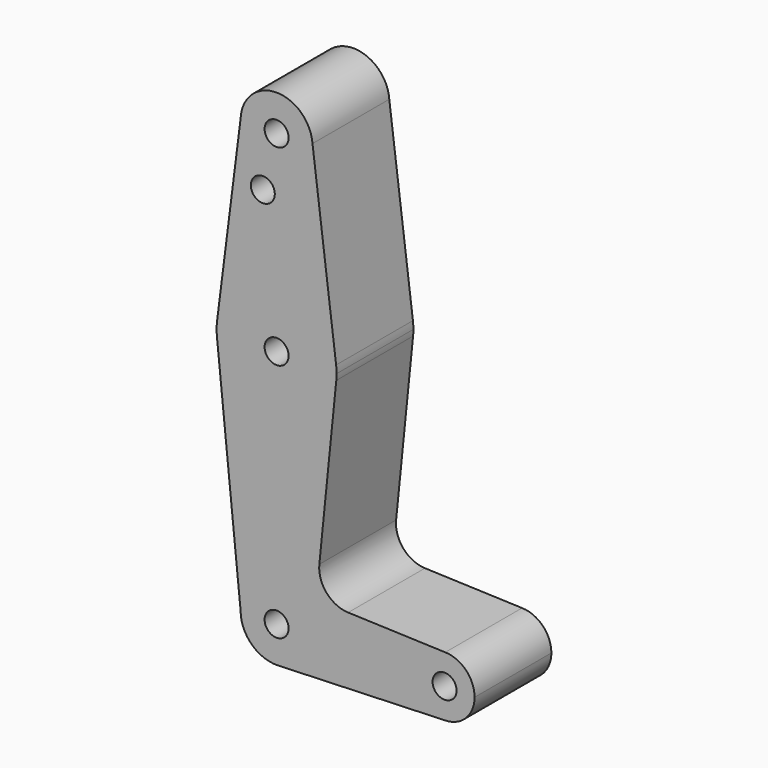
from build123d import *

# Parameters (mm, degrees)
F0_R     = 3.175
F1_DEPTH = 25.4


# Not quite as in the source:
# - a feature names something its author has since deleted; it is built from what else it names


with BuildPart() as f1:
    # F0 (on Front) → F1 (new body)
    with BuildSketch(Plane.XZ):
        with BuildLine():
            ThreePointArc((-9.5149138168, 114.7382237551), (-0.2191699059, 104.7775218797), (9.525, 114.3))
            ThreePointArc((9.525, 114.3), (9.5183168712, 114.6567477241), (9.4982768633, 115.0129948306))
            ThreePointArc((9.4982768633, 115.0129948306), (-0.1376371427, 123.8240055133), (-9.5149138168, 114.7382237551))
        make_face()
        with Locations((0, 114.3)):
            Circle(F0_R, mode=Mode.SUBTRACT)
        with BuildLine():
            ThreePointArc((9.4982768633, 115.0129948306), (9.5183168712, 114.6567477241), (9.525, 114.3))
            ThreePointArc((9.525, 114.3), (-0.2191699059, 104.7775218797), (-9.5149138168, 114.7382237551))
            Line((-9.5149138168, 114.7382237551), (-15.7492887561, 65.4938727833))
            ThreePointArc((-15.7492887561, 65.4938727833), (0.002863253, 79.3749997418), (15.7500069708, 65.4881914948))
            Line((15.7500069708, 65.4881914948), (9.4982768633, 115.0129948306))
        make_face()
        with Locations((-3.6479982082, 100.0252)):
            Circle(F0_R, mode=Mode.SUBTRACT)
        with BuildLine():
            ThreePointArc((15.875, 63.5), (15.8437209276, 64.4960583162), (15.7500069708, 65.4881914948))
            ThreePointArc((15.7500069708, 65.4881914948), (0.002863253, 79.3749997418), (-15.7492887561, 65.4938727833))
            ThreePointArc((-15.7492887561, 65.4938727833), (-15.8737601653, 63.698401651), (-15.7942028036, 61.9003804205))
            ThreePointArc((-15.7942028036, 61.9003804205), (0, 47.625), (15.7942028036, 61.9003804205))
            ThreePointArc((15.7942028036, 61.9003804205), (15.8547878338, 62.6991705884), (15.875, 63.5))
        make_face()
        with Locations((0, 63.5)):
            Circle(F0_R, mode=Mode.SUBTRACT)
        with BuildLine():
            ThreePointArc((15.7942028036, 61.9003804205), (0, 47.625), (-15.7942028036, 61.9003804205))
            Line((-15.7942028036, 61.9003804205), (-9.525, 0))
            ThreePointArc((-9.525, 0), (0, 9.525), (9.525, 0))
            ThreePointArc((9.525, 0), (6.854575784, -6.6136537422), (0.3406607199, -9.5189062016))
            Line((0.3406607199, -9.5189062016), (44.5449382907, -7.9369322141))
            ThreePointArc((44.5449382907, -7.9369322141), (36.5126173213, 0.0431562547), (44.6312377373, 7.9354306205))
            Line((44.6312377373, 7.9354306205), (18.9332319933, 8.8541850706))
            ThreePointArc((18.9332319933, 8.8541850706), (13.2249062601, 11.5746494613), (11.3075490968, 17.6003984343))
            Line((11.3075490968, 17.6003984343), (15.7942028036, 61.9003804205))
        make_face()
        with BuildLine():
            ThreePointArc((9.525, 0), (0, 9.525), (-9.525, 0))
            ThreePointArc((-9.525, 0), (-6.6136537422, -6.854575784), (0.3406607199, -9.5189062016))
            ThreePointArc((0.3406607199, -9.5189062016), (6.854575784, -6.6136537422), (9.525, 0))
        make_face()
        Circle(F0_R, mode=Mode.SUBTRACT)
        with BuildLine():
            ThreePointArc((44.6312377373, 7.9354306205), (36.5126173213, 0.0431562547), (44.5449382907, -7.9369322141))
            ThreePointArc((44.5449382907, -7.9369322141), (50.0961260583, -5.5789933486), (52.3875, 0))
            ThreePointArc((52.3875, 0), (50.126375639, 5.5482128524), (44.6312377373, 7.9354306205))
        make_face()
        with Locations((44.45, 0)):
            Circle(F0_R, mode=Mode.SUBTRACT)
    extrude(amount=F1_DEPTH)


solid = f1.part
